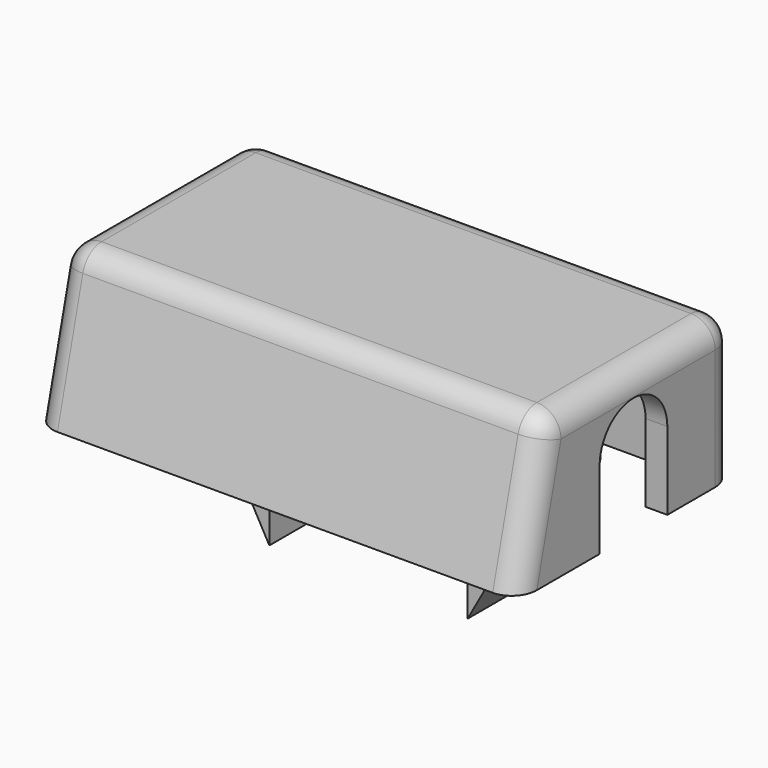
from build123d import *

# Parameters (mm, degrees)
F0_W      = 40
F0_H      = 22.5
F1_DEPTH  = 12
F3_DEPTH  = 40
F4_T      = -1.8
F6_E4_W   = 14.5
F6_E4_H   = 19.2
F7_DEPTH  = 3.6
F8_E5_W   = 14.5
F8_E5_H   = 19.2
F9_DEPTH  = 3.6
F10_W     = 5.25
F10_H     = 9
F11_DEPTH = 3.7
F12_W     = 5.25
F12_H     = 9
F13_DEPTH = 3.7
F14_W     = 1.5
F14_H     = 9
F15_DEPTH = 3.6
F16_W     = 1.5
F16_H     = 9
F17_DEPTH = 3.6
F18_W     = 7.75
F18_H     = 2.5
F19_DEPTH = 1.8
F20_W     = 7.75
F20_H     = 2.5
F21_DEPTH = 1.8
F23_DEPTH = 7.75
F25_DEPTH = 7.75
F27_DEPTH = 1.8
F29_DEPTH = 1.8
F30_R     = 2


with BuildPart() as f1:
    # F0 (on Top) → F1 (new body)
    with BuildSketch(Plane.XY):
        with Locations((-2.1441839635, 2.8779831225)):
            Rectangle(F0_W, F0_H)
    extrude(amount=F1_DEPTH)

    # F2 (on face) → F3 (cut)
    with BuildSketch(Plane.YZ.offset(17.8558160365)):
        Polygon((-8.3720168775, 12), (-8.3720168775, 0), (-5.3720168775, 12), align=None)
    extrude(amount=-F3_DEPTH, mode=Mode.SUBTRACT)

    # F4
    f4_openings = [f1.faces().sort_by_distance(p)[0] for p in [
        (-2.144184, 2.877983, 0),
    ]]
    offset(amount=F4_T, openings=f4_openings)

    # F6_E4 (on explicit) → F7 (join)
    with BuildSketch(Plane(origin=(-10.3441839635, -3.966619346, 10.2), x_dir=(0, 1, 0), z_dir=(-1, 0, 0))):
        with Locations((7.25, 9.6)):
            Rectangle(F6_E4_W, F6_E4_H)
    extrude(amount=F7_DEPTH)

    # F8_E5 (on explicit) → F9 (join)
    with BuildSketch(Plane(origin=(6.0558160365, -3.966619346, 10.2), x_dir=(0, 1, 0), z_dir=(-1, 0, 0))):
        with Locations((7.25, 9.6)):
            Rectangle(F8_E5_W, F8_E5_H)
    extrude(amount=-F9_DEPTH)

    # F10 (on face) → F11 (cut)
    with BuildSketch(Plane.YZ.offset(9.6558160365)):
        with Locations((-1.341619346, -4.5)):
            Rectangle(F10_W, F10_H)
    extrude(amount=-F11_DEPTH, mode=Mode.SUBTRACT)

    # F12 (on face) → F13 (cut)
    with BuildSketch(Plane(origin=(-13.9441839635, 0, 0), x_dir=(0, -1, 0), z_dir=(-1, 0, 0))):
        with Locations((1.341619346, -4.5)):
            Rectangle(F12_W, F12_H)
    extrude(amount=-F13_DEPTH, mode=Mode.SUBTRACT)

    # F14 (on face) → F15 (cut)
    with BuildSketch(Plane.YZ.offset(9.6558160365)):
        with Locations((9.783380654, -4.5)):
            Rectangle(F14_W, F14_H)
    extrude(amount=-F15_DEPTH, mode=Mode.SUBTRACT)

    # F16 (on face) → F17 (cut)
    with BuildSketch(Plane(origin=(-13.9441839635, 0, 0), x_dir=(0, -1, 0), z_dir=(-1, 0, 0))):
        with Locations((-9.783380654, -4.5)):
            Rectangle(F16_W, F16_H)
    extrude(amount=-F17_DEPTH, mode=Mode.SUBTRACT)

    # F18 (on face) → F19 (cut)
    with BuildSketch(Plane(origin=(-13.9441839635, 0, 0), x_dir=(0, -1, 0), z_dir=(-1, 0, 0))):
        with Locations((-5.158380654, -1.25)):
            Rectangle(F18_W, F18_H)
    extrude(amount=-F19_DEPTH, mode=Mode.SUBTRACT)

    # F20 (on face) → F21 (cut)
    with BuildSketch(Plane.YZ.offset(9.6558160365)):
        with Locations((5.158380654, -1.25)):
            Rectangle(F20_W, F20_H)
    extrude(amount=-F21_DEPTH, mode=Mode.SUBTRACT)

    # F22 (on face) → F23 (cut)
    with BuildSketch(Plane(origin=(0, 9.033380654, 0), x_dir=(-1, 0, 0), z_dir=(0, 1, 0))):
        Polygon((-6.0558160365, -9), (-9.6558160365, -2.5), (-9.6558160365, -9), align=None)
    extrude(amount=-F23_DEPTH, mode=Mode.SUBTRACT)

    # F24 (on face) → F25 (cut)
    with BuildSketch(Plane(origin=(0, 9.033380654, 0), x_dir=(-1, 0, 0), z_dir=(0, 1, 0))):
        Polygon((13.9441839635, -9), (13.9441839635, -2.5), (10.3441839635, -9), align=None)
    extrude(amount=-F25_DEPTH, mode=Mode.SUBTRACT)

    # F26 (on face) → F27 (cut)
    with BuildSketch(Plane(origin=(-22.1441839635, 0, 0), x_dir=(0, -1, 0), z_dir=(-1, 0, 0))):
        with BuildLine():
            Line((-0.1815545511, 0), (-0.1815545511, 6.4285714286))
            ThreePointArc((-0.1815545511, 6.4285714286), (-3.6815545511, 2.9285714286), (-7.1815545511, 6.4285714286))
            Line((-7.1815545511, 6.4285714286), (-7.1815545511, 0))
            Line((-7.1815545511, 0), (-0.1815545511, 0))
        make_face()
        with BuildLine():
            ThreePointArc((-7.1815545511, 6.4285714286), (-3.6815545511, 2.9285714286), (-0.1815545511, 6.4285714286))
            ThreePointArc((-0.1815545511, 6.4285714286), (-3.6815545511, 9.9285714286), (-7.1815545511, 6.4285714286))
        make_face()
    extrude(amount=-F27_DEPTH, mode=Mode.SUBTRACT)

    # F28 (on face) → F29 (cut)
    with BuildSketch(Plane.YZ.offset(17.8558160365)):
        with BuildLine():
            ThreePointArc((0.1815545511, 6.4285714286), (3.6815545511, 2.9285714286), (7.1815545511, 6.4285714286))
            ThreePointArc((7.1815545511, 6.4285714286), (3.6815545511, 9.9285714286), (0.1815545511, 6.4285714286))
        make_face()
        with BuildLine():
            Line((7.1815545511, 0), (7.1815545511, 6.4285714286))
            ThreePointArc((7.1815545511, 6.4285714286), (3.6815545511, 2.9285714286), (0.1815545511, 6.4285714286))
            Line((0.1815545511, 6.4285714286), (0.1815545511, 0))
            Line((0.1815545511, 0), (7.1815545511, 0))
        make_face()
    extrude(amount=-F29_DEPTH, mode=Mode.SUBTRACT)

    # F30
    f30_edges = [f1.edges().sort_by_distance(p)[0] for p in [
        (17.855816, -6.872017, 6),
        (17.855816, 14.127983, 6),
        (17.855816, 4.377983, 12),
        (-22.144184, -6.872017, 6),
        (-22.144184, 14.127983, 6),
        (-22.144184, 4.377983, 12),
        (-2.144184, -5.372017, 12),
        (-2.144184, 14.127983, 12),
    ]]
    fillet(f30_edges, radius=F30_R)


solid = f1.part
